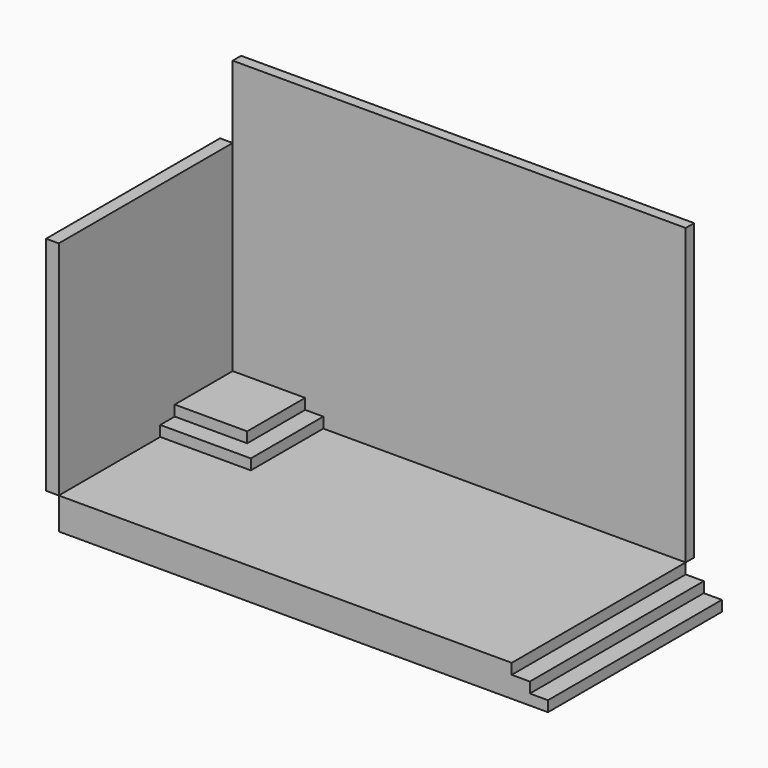
from build123d import *

# Parameters (mm, degrees)
F0_W      = 7620
F0_H      = 3657.6
F1_DEPTH  = 533.4
F2_W      = 7620
F2_H      = 3657.6
F2_W_2    = 609.6
F3_DEPTH  = 177.8
F4_W      = 1219.2
F4_H      = 1219.2
F5_DEPTH  = 355.6
F6_W      = 1524
F6_H      = 1524
F7_DEPTH  = 711.2
F9_DEPTH  = 177.8
F11_DEPTH = 213.36
F12_W     = 304.8
F12_H     = 3657.6
F13_DEPTH = 177.8


with BuildPart() as f1:
    # F0 (on Top) → F1 (new body)
    with BuildSketch(Plane.XY):
        Rectangle(F0_W, F0_H)
    extrude(amount=F1_DEPTH)

    # F2 (on face) → F3 (join)
    with BuildSketch(Plane(origin=(0, 0, 0), x_dir=(1, 0, 0), z_dir=(0, 0, -1))):
        Rectangle(F2_W, F2_H)
        with Locations((4114.8, 0)):
            Rectangle(F2_W_2, F2_H)
    extrude(amount=-F3_DEPTH)

    # F4 (on face) → F5 (join)
    with BuildSketch(Plane.XY.offset(533.4)):
        with Locations((-3200.4, 1219.2)):
            Rectangle(F4_W, F4_H)
    extrude(amount=F5_DEPTH)

    # F6 (on face) → F7 (join)
    with BuildSketch(Plane(origin=(0, 0, 0), x_dir=(1, 0, 0), z_dir=(0, 0, -1))):
        with Locations((-3048, -1066.8)):
            Rectangle(F6_W, F6_H)
    extrude(amount=-F7_DEPTH)

    # F12 (on face) → F13 (join)
    with BuildSketch(Plane.XY.offset(177.8)):
        with Locations((3962.4, 0)):
            Rectangle(F12_W, F12_H)
    extrude(amount=F13_DEPTH)


with BuildPart() as f9:
    # F8 (on face) → F9 (new body)
    with BuildSketch(Plane(origin=(0, 1828.8, 0), x_dir=(-1, 0, 0), z_dir=(0, 1, 0))):
        Polygon((2590.8, 889), (3810, 889), (3810, 5486.4), (-3810, 5486.4), (-3810, 533.4), (2286, 533.4), (2286, 711.2), (2590.8, 711.2), align=None)
    extrude(amount=F9_DEPTH)


with BuildPart() as f11:
    # F10 (on face) → F11 (new body)
    with BuildSketch(Plane(origin=(-3810, 0, 0), x_dir=(0, -1, 0), z_dir=(-1, 0, 0))):
        Polygon((-1828.8, 4267.2), (-1828.8, 889), (-609.6, 889), (-609.6, 711.2), (-304.8, 711.2), (-304.8, 533.4), (1828.8, 533.4), (1828.8, 4267.2), align=None)
    extrude(amount=F11_DEPTH)


solid = Compound([f1.part, f9.part, f11.part])
